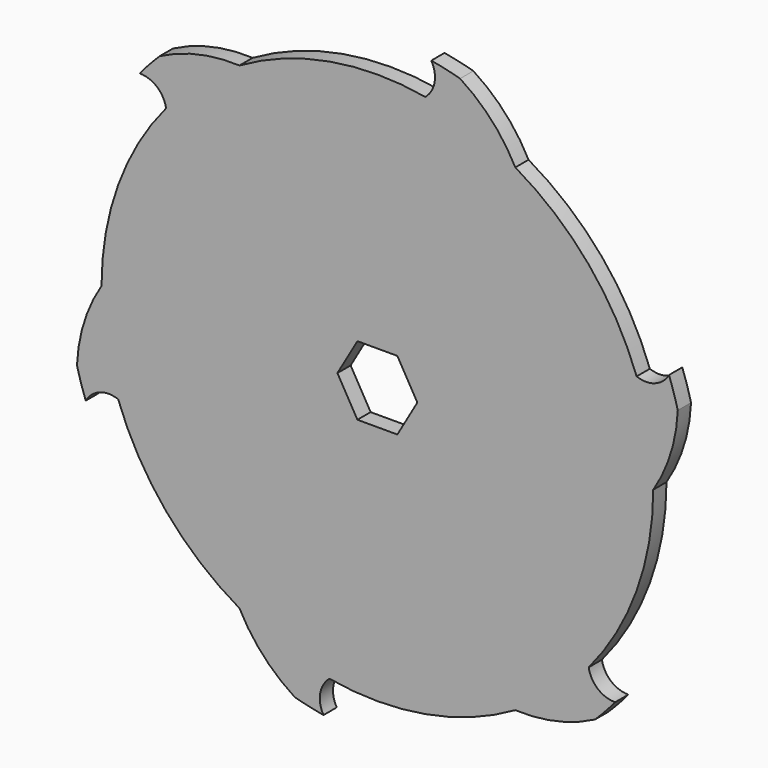
from build123d import *

# Parameters (mm, degrees)
F0_R            = 50.00625
F1_DEPTH        = 1.3335
F3_DEPTH        = 25.4
F3_DEPTH_BACK   = 25.4
F3_COPIES_COUNT = 6


# Not quite as in the source:
# - a pattern or mirror of a feature is missing from the dataset's text; its kind, count and spacing are read off the source's solid


with BuildPart() as f1:
    # F0 (on Front) → F1 (new body, symmetric)
    with BuildSketch(Plane.XZ):
        Circle(F0_R)
        Polygon((-6.4378019116, 0), (-3.2189009558, 5.5753), (3.2189009558, 5.5753), (6.4378019116, 0), (3.2189009558, -5.5753), (-3.2189009558, -5.5753), align=None, mode=Mode.SUBTRACT)
    extrude(amount=F1_DEPTH, both=True)

    # F2 (on Front) → F3 (cut, two sides)
    with BuildSketch(Plane.XZ) as f3_sk:
        with BuildLine():
            ThreePointArc((-22.225, 38.4948291982), (-7.7186614973, 43.7747046214), (7.7186614973, 43.7747046214))
            ThreePointArc((7.7186614973, 43.7747046214), (9.2172445027, 46.3314460609), (8.6834941845, 49.2465426991))
            ThreePointArc((8.6834941845, 49.2465426991), (-14.846099413, 47.7516321321), (-35.0754788107, 35.6417707931))
            ThreePointArc((-35.0754788107, 35.6417707931), (-28.8382729771, 37.9152232221), (-22.225, 38.4948291982))
        make_face()
    f3 = extrude(amount=-F3_DEPTH, mode=Mode.SUBTRACT) + extrude(f3_sk.sketch, amount=F3_DEPTH_BACK, mode=Mode.SUBTRACT)

    # F3_copies: F3 ×6 about axis
    f3_copies_axis = Axis((0, 0, 0), (0, 1, 0))
    for i in range(1, F3_COPIES_COUNT):
        add(f3.rotate(f3_copies_axis, i * 360 / F3_COPIES_COUNT), mode=Mode.SUBTRACT)


solid = f1.part
